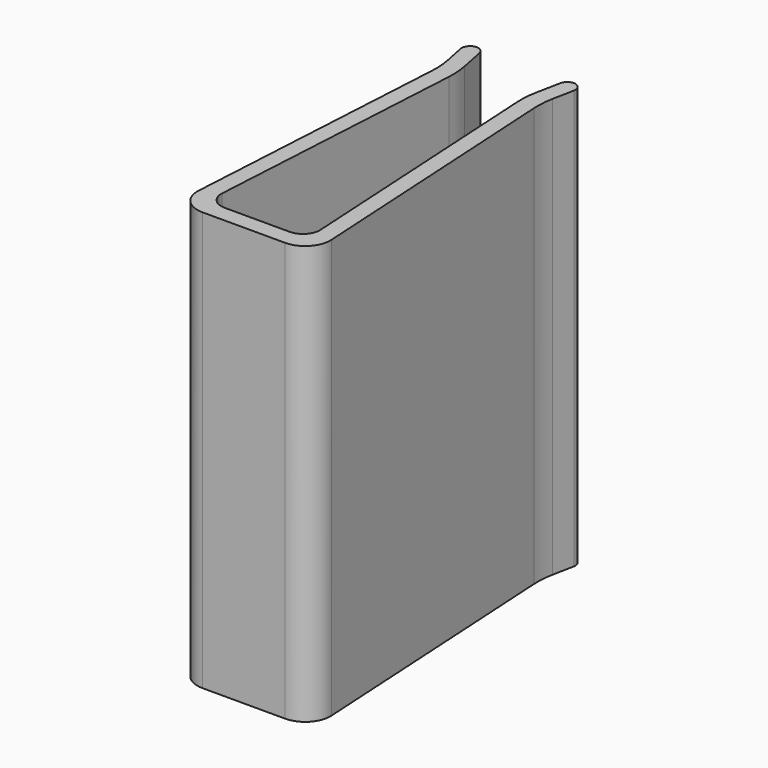
from build123d import *

# Parameters (mm, degrees)
F1_DEPTH    = 50
F3_R        = 2
F4_R        = 3
F5_R        = 2
F6_R        = 3
F7_T1_DEPTH = 54.0990195136
F7_T3_DEPTH = 56.0990195136
F8_R        = 10


# Not quite as in the source:
# - a fillet or chamfer that OpenCascade refuses, or shapes differently, is made with other operations: its cross-section is extruded or revolved along the edge and cut away or added


with BuildPart() as f1:
    # F0 (on Top) → F1 (new body)
    with BuildSketch(Plane.XY):
        Polygon((6, 0), (0, 0), (0, -2), (8.1142857143, -2), (6, 35), (7, 40), (5, 40), (4, 35), align=None)
    extrude(amount=F1_DEPTH)

    # F2: F1 across face


with BuildPart() as f1_1:
    add(f1.part)
    add(f1.part.mirror(Plane(origin=(0, -1, 25), x_dir=(0, -1, 0), z_dir=(-1, 0, 0))))

    # F3
    f3_edges = [f1_1.edges().sort_by_distance(p)[0] for p in [
        (6, 0, 25),
    ]]
    fillet(f3_edges, radius=F3_R)

    # F4
    f4_edges = [f1_1.edges().sort_by_distance(p)[0] for p in [
        (8.114286, -2, 25),
    ]]
    fillet(f4_edges, radius=F4_R)

    # F5
    f5_edges = [f1_1.edges().sort_by_distance(p)[0] for p in [
        (-6, 0, 25),
    ]]
    fillet(f5_edges, radius=F5_R)

    # F6
    f6_edges = [f1_1.edges().sort_by_distance(p)[0] for p in [
        (-8.114286, -2, 25),
    ]]
    fillet(f6_edges, radius=F6_R)

    # F7: fillet of radius 1 on 4 edges, made by hand

    # F7_s2 → F7_t1 (cut)
    with BuildSketch(Plane.XY.offset(-2.0495097568)):
        with BuildLine():
            ThreePointArc((-5.8198039027, 40), (-5.1858149971, 39.7733421413), (-4.839223227, 39.1961161351))
            Line((-4.839223227, 39.1961161351), (-5, 40))
            Line((-5, 40), (-5.8198039027, 40))
        make_face()
        with BuildLine():
            ThreePointArc((5.8198039027, 40), (5.1858149971, 39.7733421413), (4.839223227, 39.1961161351))
            Line((4.839223227, 39.1961161351), (5, 40))
            Line((5, 40), (5.8198039027, 40))
        make_face()
    extrude(amount=F7_T1_DEPTH, mode=Mode.SUBTRACT)

    # F7_s4 → F7_t3 (cut)
    with BuildSketch(Plane.XY.offset(-3.0495097568)):
        with BuildLine():
            ThreePointArc((-6.760776773, 38.8038838649), (-6.5535382386, 39.6339889056), (-5.7801960973, 40))
            Line((-5.7801960973, 40), (-7, 40))
            Line((-7, 40), (-6.760776773, 38.8038838649))
        make_face()
        with BuildLine():
            ThreePointArc((6.760776773, 38.8038838649), (6.5535382386, 39.6339889056), (5.7801960973, 40))
            Line((5.7801960973, 40), (7, 40))
            Line((7, 40), (6.760776773, 38.8038838649))
        make_face()
    extrude(amount=F7_T3_DEPTH, mode=Mode.SUBTRACT)

    # F8
    f8_edges = [f1_1.edges().sort_by_distance(p)[0] for p in [
        (-4, 35, 25),
        (4, 35, 25),
        (6, 35, 25),
        (-6, 35, 25),
    ]]
    fillet(f8_edges, radius=F8_R)


solid = f1_1.part
